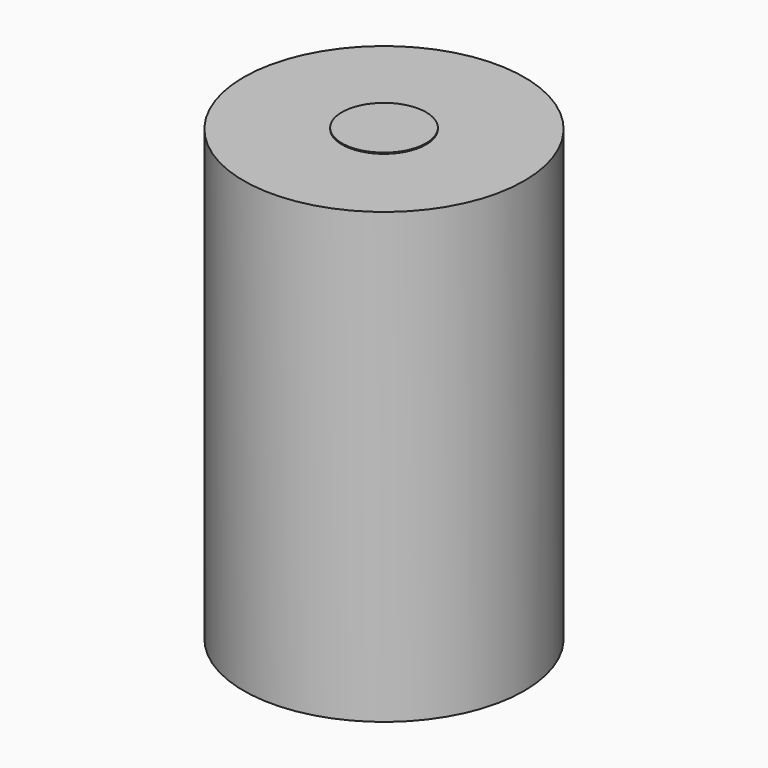
from build123d import *

# Parameters (mm, degrees)
F0_R     = 7.9375
F1_DEPTH = 25.4
F4_D     = 4.0386
F4_DEPTH = 9.525
F4_TIP   = 1.213317848
F2_R     = 2.38125
F5_DEPTH = 0.0635


# Not quite as in the source:
# - a length typed as a fraction of an inch, garbled in the dataset ("3 / 203.2 mm" for 3/8 in), is restored


with BuildPart() as f1:
    # F0 (on Top) → F1 (new body)
    with BuildSketch(Plane.XY):
        Circle(F0_R)
    extrude(amount=F1_DEPTH)

    # F4
    with Locations(Plane(origin=(0, 0, 0), x_dir=(1, 0, 0), z_dir=(0, 0, -1))):
        with Locations((0, 0)):
            Hole(F4_D / 2, depth=F4_DEPTH)
            with Locations((0, 0, -(F4_DEPTH + F4_TIP / 2))):  # 118° drill point
                Cone(0, F4_D / 2, F4_TIP, mode=Mode.SUBTRACT)

    # F2 (on face) → F5 (join)
    with BuildSketch(Plane.XY.offset(25.4)):
        Circle(F2_R)
    extrude(amount=F5_DEPTH)


solid = f1.part
